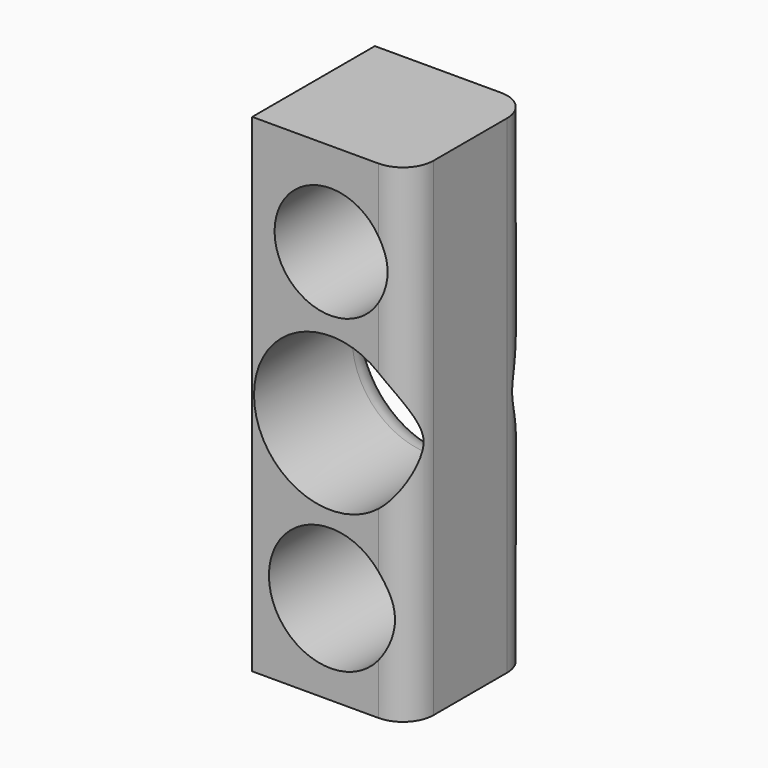
from build123d import *

# Parameters (mm, degrees)
F2_W        = 25.9886477143
F2_H        = 80.8860212564
F2_R        = 10.2254684018
F2_R_2      = 9.290469056
F3_DEPTH    = 25.4
F4_D        = 25.4
F5_T1_DEPTH = 106.2860212564


# Not quite as in the source:
# - a fillet or chamfer that OpenCascade refuses, or shapes differently, is made with other operations: its cross-section is extruded or revolved along the edge and cut away or added
# - a feature names something its author has since deleted; it is built from what else it names


with BuildPart() as f3:
    # F2 (on face) → F3 (new body)
    with BuildSketch(Plane.XZ):
        Rectangle(F2_W, F2_H)
        with Locations((0, -25.5506392568)):
            Circle(F2_R, mode=Mode.SUBTRACT)
        with Locations((0, 24.9666236341)):
            Circle(F2_R_2, mode=Mode.SUBTRACT)
    extrude(amount=F3_DEPTH)

    # F4 (through all)
    with Locations(Plane(origin=(0, 0, 0), x_dir=(1, 0, 0), z_dir=(0, 1, 0))):
        with Locations((0, 0)):
            Hole(F4_D / 2)

    # F5: fillet of radius 5.08 on 3 edges, made by hand

    # F5_s2 → F5_t1 (cut)
    with BuildSketch(Plane.XY.offset(-53.1430106282)):
        with BuildLine():
            ThreePointArc((7.9143238571, 0), (11.5064263056, -1.4878975516), (12.9943238571, -5.08))
            Line((12.9943238571, -5.08), (12.9943238571, 0))
            Line((12.9943238571, 0), (7.9143238571, 0))
        make_face()
        with BuildLine():
            ThreePointArc((7.9143238571, -25.4), (11.5064263056, -23.9121024484), (12.9943238571, -20.32))
            Line((12.9943238571, -20.32), (12.9943238571, -25.4))
            Line((12.9943238571, -25.4), (7.9143238571, -25.4))
        make_face()
    extrude(amount=F5_T1_DEPTH, mode=Mode.SUBTRACT)

    # F5_s3 → F5_t4 (revolve, cut)
    with BuildSketch(Plane.XY):
        with BuildLine():
            ThreePointArc((17.78, 0), (14.1878975516, -1.4878975516), (12.7, -5.08))
            Line((12.7, -5.08), (12.7, 0))
            Line((12.7, 0), (17.78, 0))
        make_face()
    revolve(axis=Axis((0, 0, 0), (0, 1, 0)), mode=Mode.SUBTRACT)


solid = f3.part
